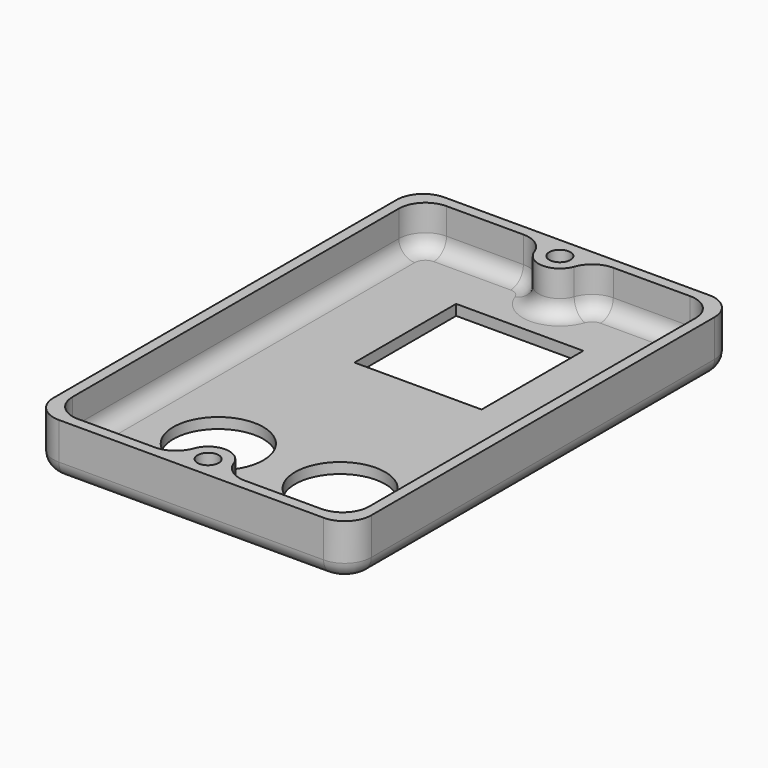
from build123d import *

# Parameters (mm, degrees)
F3_W          = 60
F3_H          = 91
F4_DEPTH      = 10
F5_W          = 56
F5_H          = 87
F5_W_2        = 24
F5_H_2        = 24
F6_DEPTH      = 8
F7_R          = 4
F8_DEPTH      = 10
F9_R          = 2
F10_DEPTH     = 10.001
F11_R         = 5
F12_R         = 5
F13_T1_DEPTH  = 77
F13_T3_DEPTH  = 14.5147186258
F13_T5_DEPTH  = 14.5147186258
F13_T8_ANGLE  = 90
F13_T10_ANGLE = 70.5287793655
F13_T12_ANGLE = 141.057558731
F13_T14_ANGLE = 90
F13_T16_ANGLE = 70.5287793655
F13_T18_ANGLE = 70.5287793655
F13_T20_ANGLE = 90
F13_T22_ANGLE = 141.057558731
F13_T24_ANGLE = 70.5287793655
F13_T26_ANGLE = 90
F13_T27_DEPTH = 81
F13_T29_DEPTH = 50
F13_T32_ANGLE = 90
F13_T34_ANGLE = 90
F13_T36_ANGLE = 90
F13_T38_ANGLE = 90
F14_R         = 8.5
F15_DEPTH     = 2.0010001
F16_DEPTH     = 10.0010001


# Not quite as in the source:
# - a fillet or chamfer that OpenCascade refuses, or shapes differently, is made with other operations: its cross-section is extruded or revolved along the edge and cut away or added


with BuildPart() as f4:
    # F3 (on Top) → F4 (new body)
    with BuildSketch(Plane.XY):
        Rectangle(F3_W, F3_H)
    extrude(amount=F4_DEPTH)

    # F5 (on face) → F6 (cut)
    with BuildSketch(Plane.XY.offset(10)):
        Rectangle(F5_W, F5_H)
        with Locations((0, 20.0242325664)):
            Rectangle(F5_W_2, F5_H_2, mode=Mode.SUBTRACT)
    extrude(amount=-F6_DEPTH, mode=Mode.SUBTRACT)

    # F7 (on face) → F8 (join)
    with BuildSketch(Plane(origin=(0, 0, 0), x_dir=(1, 0, 0), z_dir=(0, 0, -1))):
        with Locations((0, -41.5)):
            Circle(F7_R)
        with Locations((0, 41.5)):
            Circle(F7_R)
    extrude(amount=-F8_DEPTH)

    # F9 (on face) → F10 (cut, through all)
    with BuildSketch(Plane(origin=(0, 0, 0), x_dir=(1, 0, 0), z_dir=(0, 0, -1))):
        with Locations((0, -41.5)):
            Circle(F9_R)
        with Locations((0, 41.5)):
            Circle(F9_R)
    extrude(amount=-F10_DEPTH, mode=Mode.SUBTRACT)

    # F11
    f11_edges = [f4.edges().sort_by_distance(p)[0] for p in [
        (3.464102, 43.5, 6),
        (-3.464102, 43.5, 6),
        (-3.464102, -43.5, 6),
        (3.464102, -43.5, 6),
    ]]
    fillet(f11_edges, radius=F11_R)

    # F12
    f12_edges = [f4.edges().sort_by_distance(p)[0] for p in [
        (30, -45.5, 5),
        (-30, -45.5, 5),
        (30, 45.5, 5),
        (-30, 45.5, 5),
        (28, -43.5, 6),
        (-28, -43.5, 6),
        (-28, 43.5, 6),
        (28, 43.5, 6),
    ]]
    fillet(f12_edges, radius=F12_R)

    # F13: fillet of radius 3 on 24 edges, made by hand

    # F13_s2 → F13_t1 (join)
    with BuildSketch(Plane.XZ.offset(-38.5)):
        with BuildLine():
            ThreePointArc((-28, 5), (-27.1213203436, 2.8786796564), (-25, 2))
            Line((-25, 2), (-28, 2))
            Line((-28, 2), (-28, 5))
        make_face()
        with BuildLine():
            ThreePointArc((28, 5), (27.1213203436, 2.8786796564), (25, 2))
            Line((25, 2), (28, 2))
            Line((28, 2), (28, 5))
        make_face()
    extrude(amount=F13_T1_DEPTH)

    # F13_s4 → F13_t3 (join)
    with BuildSketch(Plane.YZ.offset(8.4852813742)):
        with BuildLine():
            ThreePointArc((-43.5, 5), (-42.6213203436, 2.8786796564), (-40.5, 2))
            Line((-40.5, 2), (-43.5, 2))
            Line((-43.5, 2), (-43.5, 5))
        make_face()
        with BuildLine():
            ThreePointArc((43.5, 5), (42.6213203436, 2.8786796564), (40.5, 2))
            Line((40.5, 2), (43.5, 2))
            Line((43.5, 2), (43.5, 5))
        make_face()
    extrude(amount=F13_T3_DEPTH)

    # F13_s6 → F13_t5 (join)
    with BuildSketch(Plane.YZ.offset(-23)):
        with BuildLine():
            ThreePointArc((-43.5, 5), (-42.6213203436, 2.8786796564), (-40.5, 2))
            Line((-40.5, 2), (-43.5, 2))
            Line((-43.5, 2), (-43.5, 5))
        make_face()
        with BuildLine():
            ThreePointArc((43.5, 5), (42.6213203436, 2.8786796564), (40.5, 2))
            Line((40.5, 2), (43.5, 2))
            Line((43.5, 2), (43.5, 5))
        make_face()
    extrude(amount=F13_T5_DEPTH)

    # F13_s7 → F13_t8 (revolve)
    with BuildSketch(Plane.YZ.offset(23)):
        with BuildLine():
            ThreePointArc((-43.5, 5), (-42.6213203436, 2.8786796564), (-40.5, 2))
            Line((-40.5, 2), (-43.5, 2))
            Line((-43.5, 2), (-43.5, 5))
        make_face()
    revolve(axis=Axis((23, -38.5, 2), (0, 0, 1)), revolution_arc=F13_T8_ANGLE)

    # F13_s9 → F13_t10 (revolve)
    with BuildSketch(Plane.YZ.offset(8.4852813742)):
        with BuildLine():
            ThreePointArc((-43.5, 5), (-42.6213203436, 2.8786796564), (-40.5, 2))
            Line((-40.5, 2), (-43.5, 2))
            Line((-43.5, 2), (-43.5, 5))
        make_face()
    revolve(axis=Axis((8.4852813742, -38.5, 2), (0, 0, -1)), revolution_arc=F13_T10_ANGLE)

    # F13_s11 → F13_t12 (revolve)
    with BuildSketch(Plane(origin=(-13.0421917419, -36.8888888889, 0), x_dir=(0, 0, 1), z_dir=(-0.3333333333, -0.9428090416, 0))):
        with BuildLine():
            ThreePointArc((5, -9.8333333333), (2.8786796564, -8.9546536769), (2, -6.8333333333))
            Line((2, -6.8333333333), (2, -9.8333333333))
            Line((2, -9.8333333333), (5, -9.8333333333))
        make_face()
    revolve(axis=Axis((0, -41.5, 2), (0, 0, -1)), revolution_arc=F13_T12_ANGLE)

    # F13_s13 → F13_t14 (revolve)
    with BuildSketch(Plane.XZ.offset(-38.5)):
        with BuildLine():
            ThreePointArc((28, 5), (27.1213203436, 2.8786796564), (25, 2))
            Line((25, 2), (28, 2))
            Line((28, 2), (28, 5))
        make_face()
    revolve(axis=Axis((23, 38.5, 2), (0, 0, 1)), revolution_arc=F13_T14_ANGLE)

    # F13_s15 → F13_t16 (revolve)
    with BuildSketch(Plane(origin=(-13.0421917419, -36.8888888889, 0), x_dir=(0, 0, 1), z_dir=(0.3333333333, 0.9428090416, 0))):
        with BuildLine():
            ThreePointArc((5, 9.8333333333), (2.8786796564, 8.9546536769), (2, 6.8333333333))
            Line((2, 6.8333333333), (2, 9.8333333333))
            Line((2, 9.8333333333), (5, 9.8333333333))
        make_face()
    revolve(axis=Axis((-8.4852813742, -38.5, 2), (0, 0, -1)), revolution_arc=F13_T16_ANGLE)

    # F13_s17 → F13_t18 (revolve)
    with BuildSketch(Plane.YZ.offset(8.4852813742)):
        with BuildLine():
            ThreePointArc((43.5, 5), (42.6213203436, 2.8786796564), (40.5, 2))
            Line((40.5, 2), (43.5, 2))
            Line((43.5, 2), (43.5, 5))
        make_face()
    revolve(axis=Axis((8.4852813742, 38.5, 2), (0, 0, 1)), revolution_arc=F13_T18_ANGLE)

    # F13_s19 → F13_t20 (revolve)
    with BuildSketch(Plane.YZ.offset(-23)):
        with BuildLine():
            ThreePointArc((-43.5, 5), (-42.6213203436, 2.8786796564), (-40.5, 2))
            Line((-40.5, 2), (-43.5, 2))
            Line((-43.5, 2), (-43.5, 5))
        make_face()
    revolve(axis=Axis((-23, -38.5, 2), (0, 0, -1)), revolution_arc=F13_T20_ANGLE)

    # F13_s21 → F13_t22 (revolve)
    with BuildSketch(Plane(origin=(13.0421917419, 36.8888888889, 0), x_dir=(0, 0, 1), z_dir=(0.3333333333, 0.9428090416, 0))):
        with BuildLine():
            ThreePointArc((5, -9.8333333333), (2.8786796564, -8.9546536769), (2, -6.8333333333))
            Line((2, -6.8333333333), (2, -9.8333333333))
            Line((2, -9.8333333333), (5, -9.8333333333))
        make_face()
    revolve(axis=Axis((0, 41.5, 2), (0, 0, -1)), revolution_arc=F13_T22_ANGLE)

    # F13_s23 → F13_t24 (revolve)
    with BuildSketch(Plane(origin=(-13.0421917419, 36.8888888889, 0), x_dir=(0, 0, 1), z_dir=(0.3333333333, -0.9428090416, 0))):
        with BuildLine():
            ThreePointArc((5, -9.8333333333), (2.8786796564, -8.9546536769), (2, -6.8333333333))
            Line((2, -6.8333333333), (2, -9.8333333333))
            Line((2, -9.8333333333), (5, -9.8333333333))
        make_face()
    revolve(axis=Axis((-8.4852813742, 38.5, 2), (0, 0, 1)), revolution_arc=F13_T24_ANGLE)

    # F13_s25 → F13_t26 (revolve)
    with BuildSketch(Plane.XZ.offset(-38.5)):
        with BuildLine():
            ThreePointArc((-28, 5), (-27.1213203436, 2.8786796564), (-25, 2))
            Line((-25, 2), (-28, 2))
            Line((-28, 2), (-28, 5))
        make_face()
    revolve(axis=Axis((-23, 38.5, 2), (0, 0, -1)), revolution_arc=F13_T26_ANGLE)

    # F13_s28 → F13_t27 (cut)
    with BuildSketch(Plane.XZ.offset(-40.5)):
        with BuildLine():
            ThreePointArc((30, 3), (29.1213203436, 0.8786796564), (27, 0))
            Line((27, 0), (30, 0))
            Line((30, 0), (30, 3))
        make_face()
        with BuildLine():
            ThreePointArc((-30, 3), (-29.1213203436, 0.8786796564), (-27, 0))
            Line((-27, 0), (-30, 0))
            Line((-30, 0), (-30, 3))
        make_face()
    extrude(amount=F13_T27_DEPTH, mode=Mode.SUBTRACT)

    # F13_s30 → F13_t29 (cut)
    with BuildSketch(Plane.YZ.offset(-25)):
        with BuildLine():
            ThreePointArc((-45.5, 3), (-44.6213203436, 0.8786796564), (-42.5, 0))
            Line((-42.5, 0), (-45.5, 0))
            Line((-45.5, 0), (-45.5, 3))
        make_face()
        with BuildLine():
            ThreePointArc((45.5, 3), (44.6213203436, 0.8786796564), (42.5, 0))
            Line((42.5, 0), (45.5, 0))
            Line((45.5, 0), (45.5, 3))
        make_face()
    extrude(amount=F13_T29_DEPTH, mode=Mode.SUBTRACT)

    # F13_s31 → F13_t32 (revolve, cut)
    with BuildSketch(Plane.YZ.offset(25)):
        with BuildLine():
            ThreePointArc((-45.5, 3), (-44.6213203436, 0.8786796564), (-42.5, 0))
            Line((-42.5, 0), (-45.5, 0))
            Line((-45.5, 0), (-45.5, 3))
        make_face()
    revolve(axis=Axis((25, -40.5, 0), (0, 0, 1)), revolution_arc=F13_T32_ANGLE, mode=Mode.SUBTRACT)

    # F13_s33 → F13_t34 (revolve, cut)
    with BuildSketch(Plane.YZ.offset(-25)):
        with BuildLine():
            ThreePointArc((-45.5, 3), (-44.6213203436, 0.8786796564), (-42.5, 0))
            Line((-42.5, 0), (-45.5, 0))
            Line((-45.5, 0), (-45.5, 3))
        make_face()
    revolve(axis=Axis((-25, -40.5, 0), (0, 0, -1)), revolution_arc=F13_T34_ANGLE, mode=Mode.SUBTRACT)

    # F13_s35 → F13_t36 (revolve, cut)
    with BuildSketch(Plane.XZ.offset(-40.5)):
        with BuildLine():
            ThreePointArc((30, 3), (29.1213203436, 0.8786796564), (27, 0))
            Line((27, 0), (30, 0))
            Line((30, 0), (30, 3))
        make_face()
    revolve(axis=Axis((25, 40.5, 0), (0, 0, 1)), revolution_arc=F13_T36_ANGLE, mode=Mode.SUBTRACT)

    # F13_s37 → F13_t38 (revolve, cut)
    with BuildSketch(Plane.XZ.offset(-40.5)):
        with BuildLine():
            ThreePointArc((-30, 3), (-29.1213203436, 0.8786796564), (-27, 0))
            Line((-27, 0), (-30, 0))
            Line((-30, 0), (-30, 3))
        make_face()
    revolve(axis=Axis((-25, 40.5, 0), (0, 0, -1)), revolution_arc=F13_T38_ANGLE, mode=Mode.SUBTRACT)

    # F14 (on face) → F15 (cut, through all)
    with BuildSketch(Plane.XY.offset(2)):
        with Locations((11.5, -24.7238390148)):
            Circle(F14_R)
        with Locations((-11.5, -24.7238390148)):
            Circle(F14_R)
    extrude(amount=-F15_DEPTH, mode=Mode.SUBTRACT)

    # F16 (cut, through all): a face of the model
    f16_faces = [f4.faces().sort_by_distance(p)[0] for p in [
        (0, 20.0242325664, 10),
    ]]
    extrude(f16_faces, amount=-F16_DEPTH, mode=Mode.SUBTRACT)


solid = f4.part
